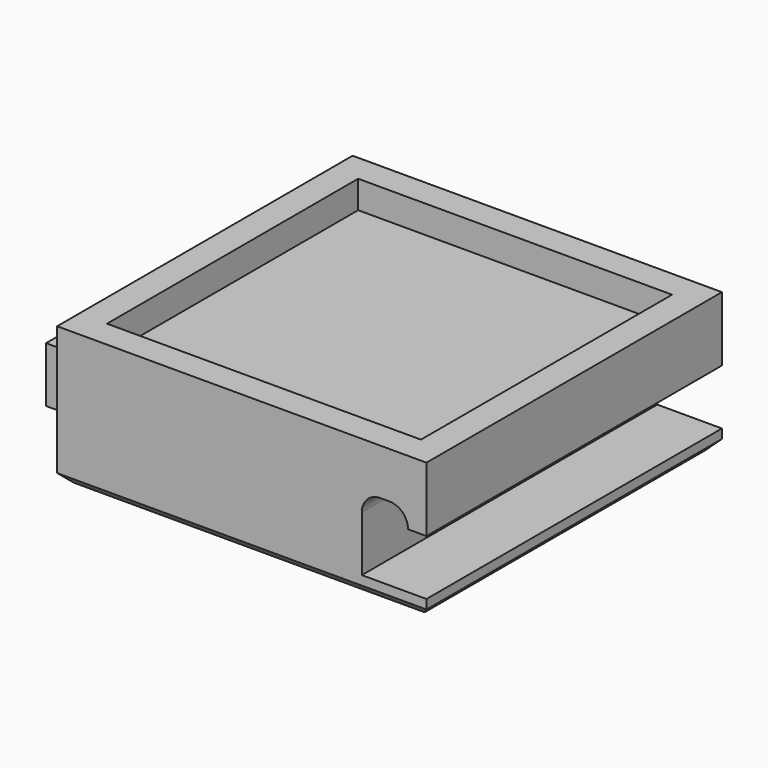
from build123d import *

# Parameters (mm, degrees)
F0_W      = 20
F0_H      = 20
F1_DEPTH  = 1.5
F2_W      = 3
F2_H      = 14
F3_DEPTH  = 1.5
F4_W      = 1.5
F4_H      = 14
F5_DEPTH  = 1.5
F6_DEPTH  = 6
F7_W      = 17
F7_H      = 17
F8_DEPTH  = 1.5
F9_W      = 2.5
F9_H      = 1
F10_DEPTH = 20
F11_R     = 0.99999
F12_R     = 0.5
F13_SIZE  = 0.5


# Not quite as in the source:
# - a fillet or chamfer is up to 0.001 mm smaller than in the source, because OpenCascade refuses the exact size


with BuildPart() as f1:
    # F0 (on Top) → F1 (new body)
    with BuildSketch(Plane.XY):
        Rectangle(F0_W, F0_H)
    extrude(amount=F1_DEPTH)

    # F6 (add): a face of the model
    f6_faces = [f1.faces().sort_by_distance(p)[0] for p in [
        (0, 0, 1.5),
    ]]


with BuildPart() as f3:
    # F2 (on face) → F3 (new body)
    with BuildSketch(Plane.XY.offset(1.5)):
        with Locations((-11.5, 0)):
            Rectangle(F2_W, F2_H)
    extrude(amount=F3_DEPTH)

    # F4 (on face) → F5 (join)
    with BuildSketch(Plane.XY.offset(3)):
        with Locations((-12.25, 0)):
            Rectangle(F4_W, F4_H)
    extrude(amount=F5_DEPTH)


with BuildPart() as f1_1:
    add(f1.part)

    add(f3.part)  # F6 merges F3
    extrude(f6_faces, amount=F6_DEPTH)

    # F7 (on face) → F8 (cut)
    with BuildSketch(Plane.XY.offset(7.5)):
        Rectangle(F7_W, F7_H)
    extrude(amount=-F8_DEPTH, mode=Mode.SUBTRACT)

    # F9 (on face) → F10 (cut, through all)
    with BuildSketch(Plane.XZ.offset(10)):
        Polygon((6.5, 1), (10, 1), (10, 4), (9, 4), (6.5, 4), align=None)
        with Locations((7.75, 4.5)):
            Rectangle(F9_W, F9_H)
    extrude(amount=-F10_DEPTH, mode=Mode.SUBTRACT)

    # F11 (radius 1 in the source; OpenCascade refuses exactly that, so slightly less here)
    f11_edges = [f1_1.edges().sort_by_distance(p)[0] for p in [
        (6.5, 0, 5),
        (9, 0, 5),
    ]]
    fillet(f11_edges, radius=F11_R)

    # F12
    f12_edges = [f1_1.edges().sort_by_distance(p)[0] for p in [
        (-10, 0, 3),
    ]]
    fillet(f12_edges, radius=F12_R)

    # F13
    f13_edges = [f1_1.edges().sort_by_distance(p)[0] for p in [
        (0, -10, 0),
        (10, 0, 0),
        (0, 10, 0),
        (-10, 0, 0),
    ]]
    chamfer(f13_edges, length=F13_SIZE)


solid = f1_1.part
